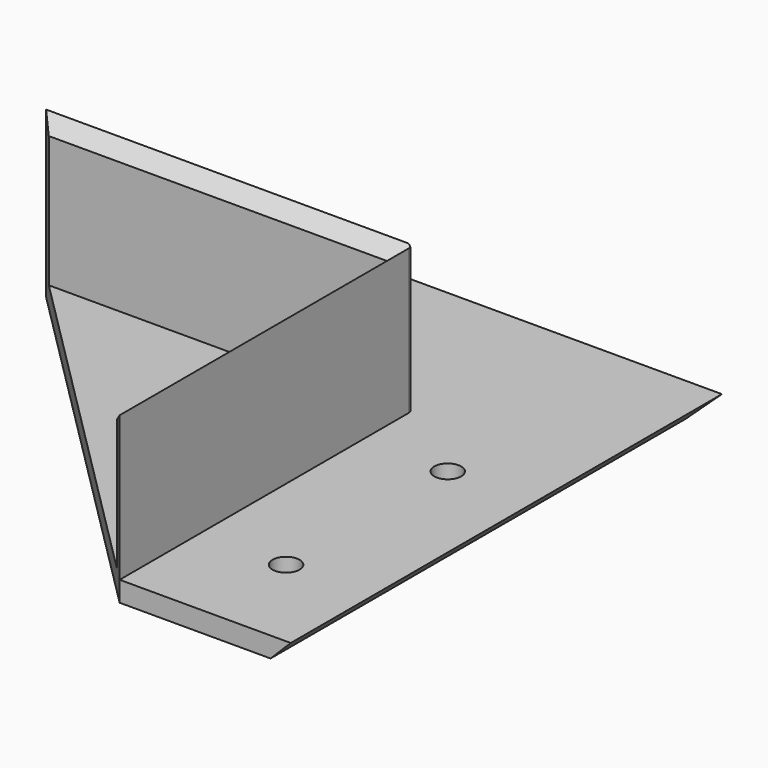
from build123d import *

# Parameters (mm, degrees)
F0_R        = 2
F1_DEPTH    = 3
F3_DEPTH    = 21.5
F4_SIZE     = 2.99999
F5_R        = 1
F6_T4_DEPTH = 60.8867319519
F6_T9_DEPTH = 60.8867319519


# Not quite as in the source:
# - a fillet or chamfer that OpenCascade refuses, or shapes differently, is made with other operations: its cross-section is extruded or revolved along the edge and cut away or added
# - a fillet or chamfer is up to 0.001 mm smaller than in the source, because OpenCascade refuses the exact size


with BuildPart() as f1:
    # F0 (on Top) → F1 (new body)
    with BuildSketch(Plane.XY):
        Polygon((0, -80), (0, 0), (-80, 0), (-80, -25.4), (-25.4, -80), align=None)
        with Locations((-12.7, -65)):
            Circle(F0_R, mode=Mode.SUBTRACT)
        with Locations((-70, -12.7)):
            Circle(F0_R, mode=Mode.SUBTRACT)
        with Locations((-12.7, -35)):
            Circle(F0_R, mode=Mode.SUBTRACT)
        with Locations((-40, -12.7)):
            Circle(F0_R, mode=Mode.SUBTRACT)
    extrude(amount=F1_DEPTH)

    # F2 (on face) → F3 (join)
    with BuildSketch(Plane.XY.offset(3)):
        Polygon((-25.4, -25.4), (-80, -25.4), (-78, -27.4), (-27.4, -27.4), (-27.4, -78), (-25.4, -80), align=None)
    extrude(amount=F3_DEPTH)

    # F4 (size 3 in the source; OpenCascade refuses exactly that, so slightly less here)
    f4_edges = [f1.edges().sort_by_distance(p)[0] for p in [
        (-40, 0, 0),
        (0, -40, 0),
    ]]
    chamfer(f4_edges, length=F4_SIZE)

    # F5
    f5_edges = [f1.edges().sort_by_distance(p)[0] for p in [
        (-25.4, -25.4, 13.75),
    ]]
    fillet(f5_edges, radius=F5_R)

    # F6: chamfer of 2 on 2 edges, made by hand


with BuildPart() as f6_tool2:
    # F6_s3 → F6_t4 (new body)
    with BuildSketch(Plane.YZ.offset(-83.1433659759)):
        Polygon((-25.4, 24.5), (-27.4, 22.5), (-27.4, 24.5), align=None)
    extrude(amount=F6_T4_DEPTH)

    split(bisect_by=Plane(origin=(-24.95, 0, 24.95), x_dir=(0, 1, 0), z_dir=(-0.7071067812, 0, 0.7071067812)), keep=Keep.TOP)


with BuildPart() as f1_1:
    add(f1.part)

    # F6_t1: cut F6_tool2
    add(f6_tool2.part, mode=Mode.SUBTRACT)


with BuildPart() as f6_tool7:
    # F6_s8 → F6_t9 (new body)
    with BuildSketch(Plane.XZ.offset(22.2566340241)):
        Polygon((-25.4, 24.5), (-27.4, 22.5), (-27.4, 24.5), align=None)
    extrude(amount=F6_T9_DEPTH)

    split(bisect_by=Plane(origin=(0, -24.95, 24.95), x_dir=(1, 0, 0), z_dir=(0, -0.7071067812, 0.7071067812)), keep=Keep.TOP)


with BuildPart() as f1_2:
    add(f1_1.part)

    # F6_t6: cut F6_tool7
    add(f6_tool7.part, mode=Mode.SUBTRACT)


solid = f1_2.part
